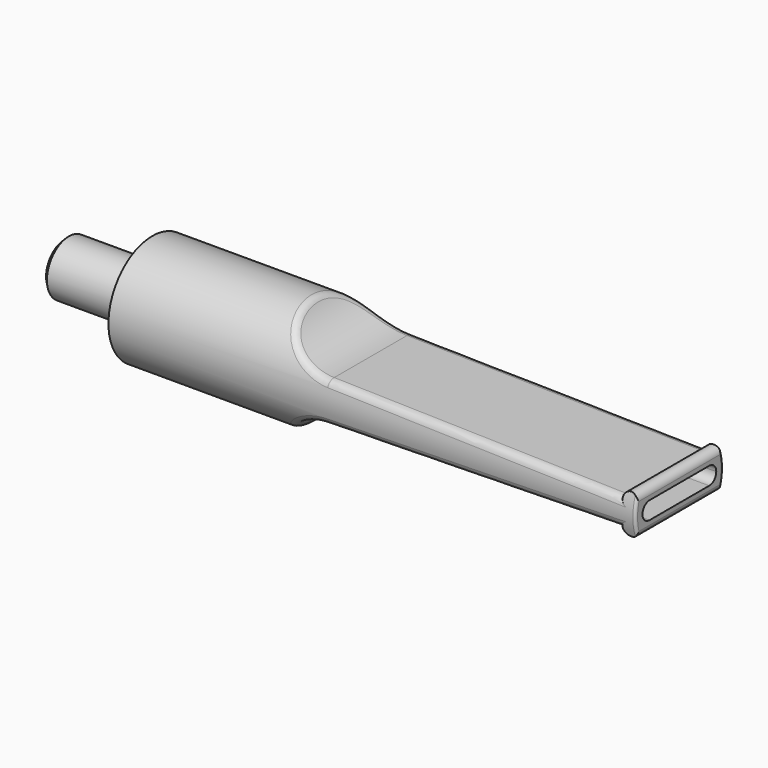
from build123d import *

# Parameters (mm, degrees)
F0_R         = 7.9375
F0_R_2       = 1.27
F1_DEPTH     = 76.2
F2_R         = 3.96875
F2_R_2       = 1.27
F3_DEPTH     = 12.7
F4_SIZE      = 0.635
F6_DEPTH     = 12.7
F7_R         = 1.143
F9_DEPTH     = 50.8
F10_T2_ANGLE = 20.7620996395
F10_T4_ANGLE = 41.5245937011
F10_T6_ANGLE = 20.7620996395


# Not quite as in the source:
# - a fillet or chamfer that OpenCascade refuses, or shapes differently, is made with other operations: its cross-section is extruded or revolved along the edge and cut away or added


with BuildPart() as f1:
    # F0 (on Right) → F1 (new body)
    with BuildSketch(Plane.YZ):
        Circle(F0_R)
        Circle(F0_R_2, mode=Mode.SUBTRACT)
    extrude(amount=F1_DEPTH)

    # F2 (on face) → F3 (join)
    with BuildSketch(Plane(origin=(0, 0, 0), x_dir=(0, -1, 0), z_dir=(-1, 0, 0))):
        Circle(F2_R)
        Circle(F2_R_2, mode=Mode.SUBTRACT)
    extrude(amount=F3_DEPTH)

    # F4
    f4_edges = [f1.edges().sort_by_distance(p)[0] for p in [
        (-12.7, 3.96875, 0),
    ]]
    chamfer(f4_edges, length=F4_SIZE)

    # F5 (on Front) → F6 (cut, symmetric)
    with BuildSketch(Plane.XZ):
        with BuildLine():
            Line((76.2, 7.9375), (23.7019209521, 7.9375))
            ThreePointArc((23.7019209521, 7.9375), (26.9034176774, 4.2751789317), (31.5531231463, 2.8460477479))
            Line((31.5531231463, 2.8460477479), (74.1756562462, 1.9476682506))
            ThreePointArc((74.1756562462, 1.9476682506), (75.207436609, 2.8566351207), (76.2, 1.905))
            Line((76.2, 1.905), (76.2, 7.9375))
        make_face()
        with BuildLine():
            Line((76.2, -7.9375), (76.2, -1.905))
            ThreePointArc((76.2, -1.905), (75.207436609, -2.8566351207), (74.1756562462, -1.9476682506))
            Line((74.1756562462, -1.9476682506), (31.5531231463, -2.8460477479))
            ThreePointArc((31.5531231463, -2.8460477479), (26.9034176774, -4.2751789317), (23.7019209521, -7.9375))
            Line((23.7019209521, -7.9375), (76.2, -7.9375))
        make_face()
    extrude(amount=F6_DEPTH, both=True, mode=Mode.SUBTRACT)

    # F7
    f7_edges = [f1.edges().sort_by_distance(p)[0] for p in [
        (52.864291, 7.566966, 2.39686),
        (52.864291, -7.566966, 2.39686),
        (52.864291, -7.566966, -2.39686),
        (52.864291, 7.566966, -2.39686),
        (23.701921, 0.000372, 7.9375),
        (23.701921, -0.000372, -7.9375),
    ]]
    fillet(f7_edges, radius=F7_R)

    # F8 (on face) → F9 (cut)
    with BuildSketch(Plane.YZ.offset(76.2)):
        with BuildLine():
            Line((5.3975, 1.27), (-5.3975, 1.27))
            ThreePointArc((-5.3975, 1.27), (-6.2955256121, 0.8980256121), (-6.6675, 0))
            ThreePointArc((-6.6675, 0), (-6.2955256121, -0.8980256121), (-5.3975, -1.27))
            Line((-5.3975, -1.27), (5.3975, -1.27))
            ThreePointArc((5.3975, -1.27), (6.2955256121, -0.8980256121), (6.6675, 0))
            ThreePointArc((6.6675, 0), (6.2955256121, 0.8980256121), (5.3975, 1.27))
        make_face()
    extrude(amount=-F9_DEPTH, mode=Mode.SUBTRACT)

    # F10: fillet of radius 0.381 on 3 edges, made by hand

    # F10_s1 → F10_t2 (revolve, cut)
    with BuildSketch(Plane.XY):
        with BuildLine():
            ThreePointArc((75.819, 7.9375), (76.0884076836, 7.8259076836), (76.2, 7.5565))
            Line((76.2, 7.5565), (76.2, 7.9375))
            Line((76.2, 7.9375), (75.819, 7.9375))
        make_face()
    revolve(axis=Axis((76.2, 0, 0), (1, 0, 0)), revolution_arc=F10_T2_ANGLE, mode=Mode.SUBTRACT)

    # F10_s3 → F10_t4 (revolve, cut)
    with BuildSketch(Plane(origin=(0, 0, 0), x_dir=(1, 0, 0), z_dir=(0, 0.3544917291, 0.93505915))):
        with BuildLine():
            ThreePointArc((75.819, -7.9375), (76.0884076836, -7.8259076836), (76.2, -7.5565))
            Line((76.2, -7.5565), (76.2, -7.9375))
            Line((76.2, -7.9375), (75.819, -7.9375))
        make_face()
    revolve(axis=Axis((76.2, 0, 0), (1, 0, 0)), revolution_arc=F10_T4_ANGLE, mode=Mode.SUBTRACT)

    # F10_s5 → F10_t6 (revolve, cut)
    with BuildSketch(Plane(origin=(0, 0, 0), x_dir=(1, 0, 0), z_dir=(0, -0.3544885106, -0.9350603702))):
        with BuildLine():
            ThreePointArc((75.819, -7.9375), (76.0884076836, -7.8259076836), (76.2, -7.5565))
            Line((76.2, -7.5565), (76.2, -7.9375))
            Line((76.2, -7.9375), (75.819, -7.9375))
        make_face()
    revolve(axis=Axis((76.2, 0, 0), (1, 0, 0)), revolution_arc=F10_T6_ANGLE, mode=Mode.SUBTRACT)


solid = f1.part
